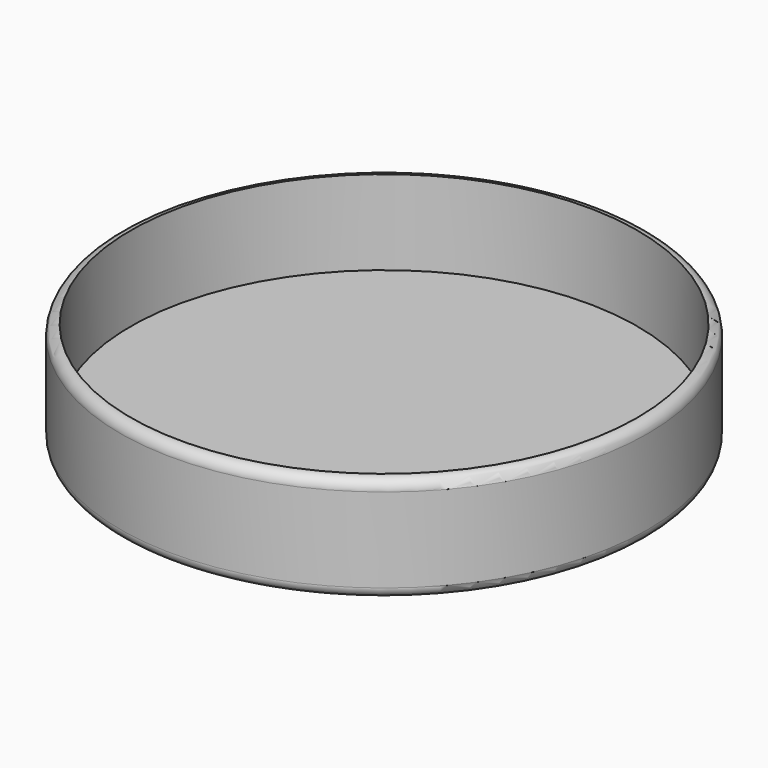
from build123d import *

# Parameters (mm, degrees)
F0_R     = 25
F1_DEPTH = 10
F2_R     = 24
F3_DEPTH = 8
F4_R     = 0.99999
F5_R     = 1


# Not quite as in the source:
# - a fillet or chamfer is up to 0.001 mm smaller than in the source, because OpenCascade refuses the exact size


with BuildPart() as f1:
    # F0 (on Top) → F1 (new body)
    with BuildSketch(Plane.XY):
        Circle(F0_R)
    extrude(amount=F1_DEPTH)

    # F2 (on face) → F3 (cut)
    with BuildSketch(Plane.XY.offset(10)):
        Circle(F2_R)
    extrude(amount=-F3_DEPTH, mode=Mode.SUBTRACT)

    # F4 (radius 1 in the source; OpenCascade refuses exactly that, so slightly less here)
    f4_edges = [f1.edges().sort_by_distance(p)[0] for p in [
        (-25, 0, 10),
    ]]
    fillet(f4_edges, radius=F4_R)

    # F5
    f5_edges = [f1.edges().sort_by_distance(p)[0] for p in [
        (-25, 0, 0),
    ]]
    fillet(f5_edges, radius=F5_R)


solid = f1.part
